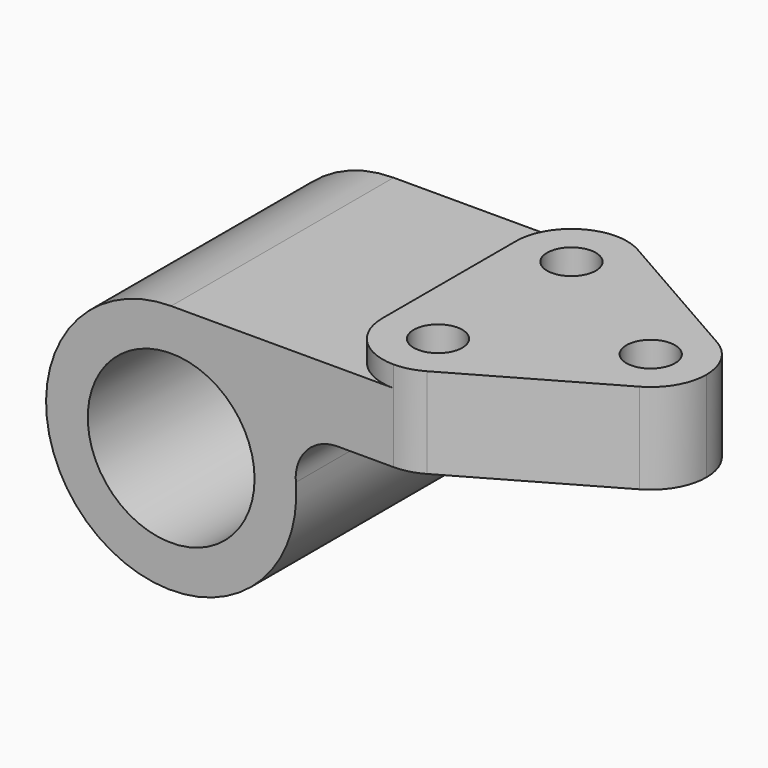
from build123d import *

# Parameters (mm, degrees)
F0_R     = 19.05
F1_DEPTH = 63.5
F2_R     = 5.5626
F3_DEPTH = 61.9262
F4_DEPTH = 4.7752
F5_DEPTH = 61.9262


with BuildPart() as f1:
    # F0 (on Front) → F1 (new body)
    with BuildSketch(Plane.XZ):
        with BuildLine():
            Line((38.1, 28.575), (0, 28.575))
            ThreePointArc((0, 28.575), (-19.345366451, -21.0306305629), (28.4756083945, 2.38125))
            ThreePointArc((28.4756083945, 2.38125), (30.9572676717, 9.6234554837), (37.9674778593, 12.7))
            Line((37.9674778593, 12.7), (96.8502, 12.7))
            Line((96.8502, 12.7), (96.8502, 33.3502))
            Line((96.8502, 33.3502), (38.1, 33.3502))
            Line((38.1, 33.3502), (38.1, 28.575))
        make_face()
        Circle(F0_R, mode=Mode.SUBTRACT)
    extrude(amount=F1_DEPTH)

    # F2 (on face) → F3 (cut, through all)
    with BuildSketch(Plane.XY.offset(33.3502)):
        with Locations((50.8, -50.8)):
            Circle(F2_R)
        with Locations((50.8, -12.7)):
            Circle(F2_R)
        with Locations((84.1502, -31.75)):
            Circle(F2_R)
    extrude(amount=-F3_DEPTH, mode=Mode.SUBTRACT)

    # F2 (on face) → F4 (cut)
    with BuildSketch(Plane.XY.offset(33.3502)):
        with BuildLine():
            ThreePointArc((38.1, -12.7), (41.8197438789, -3.7197438789), (50.8, 0))
            Line((50.8, 0), (38.1, 0))
            Line((38.1, 0), (38.1, -12.7))
        make_face()
        with BuildLine():
            Line((38.1, -63.5), (50.8, -63.5))
            ThreePointArc((50.8, -63.5), (41.8197438789, -59.7802561211), (38.1, -50.8))
            Line((38.1, -50.8), (38.1, -63.5))
        make_face()
    extrude(amount=-F4_DEPTH, mode=Mode.SUBTRACT)

    # F2 (on face) → F5 (cut, through all)
    with BuildSketch(Plane.XY.offset(33.3502)):
        with BuildLine():
            ThreePointArc((96.8502, -31.75), (95.1340352623, -38.1253715915), (90.4493554441, -42.7777214642))
            Line((90.4493554441, -42.7777214642), (57.0991554441, -61.8277214642))
            ThreePointArc((57.0991554441, -61.8277214642), (54.0586759125, -63.0748128824), (50.8, -63.5))
            Line((50.8, -63.5), (96.8502, -63.5))
            Line((96.8502, -63.5), (96.8502, -31.75))
        make_face()
        with BuildLine():
            ThreePointArc((90.4493554441, -20.7222785358), (95.1340352623, -25.3746284085), (96.8502, -31.75))
            Line((96.8502, -31.75), (96.8502, 0))
            Line((96.8502, 0), (50.8, 0))
            ThreePointArc((50.8, 0), (54.0586759125, -0.4251871176), (57.0991554441, -1.6722785358))
            Line((57.0991554441, -1.6722785358), (90.4493554441, -20.7222785358))
        make_face()
    extrude(amount=-F5_DEPTH, mode=Mode.SUBTRACT)


solid = f1.part
